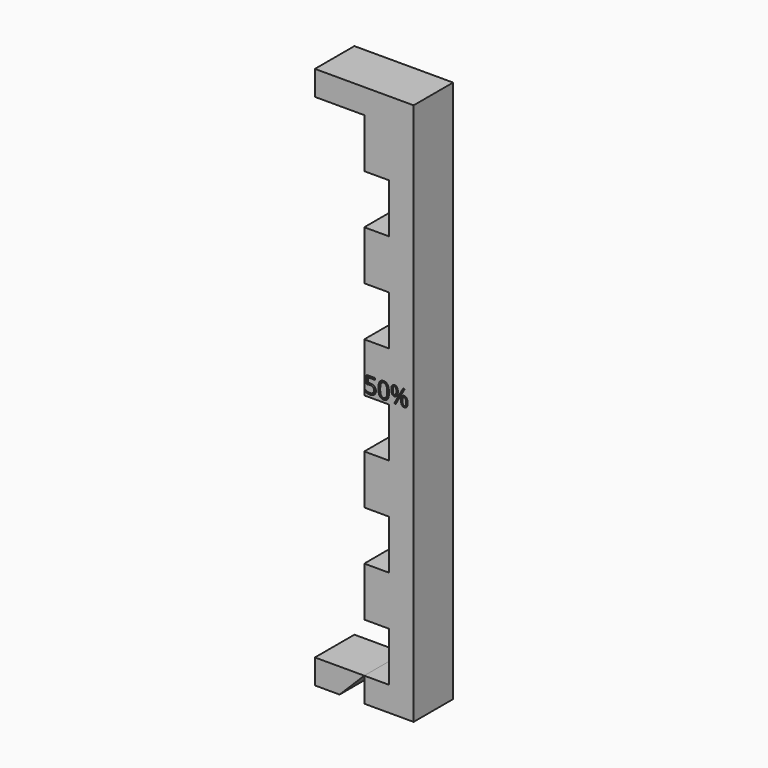
from build123d import *

# Parameters (mm, degrees)
F1_DEPTH     = 110
F2_W         = 10
F2_H         = 10
F3_DEPTH     = 5
F4_SIZE      = 4.99999
F6_DEPTH     = 10
F7_W         = 15
F7_H         = 5
F8_DEPTH     = 10
F9_TEXT_SIZE = 4.5843714191
F10_DEPTH    = 0.5
F11_SCALE    = 0.5
F12_ANGLE    = 90
F13_DEPTH    = 5


# Not quite as in the source:
# - a fillet or chamfer is up to 0.001 mm smaller than in the source, because OpenCascade refuses the exact size
# - Text() gives the source's letters only with a copy of the font that has no kerning and outlines rounded to 1/6400 em; it was checked with that copy


with BuildPart() as f1:
    # F0 (on Front) → F1 (new body)
    with BuildSketch(Plane.XZ):
        Polygon((10, 10), (0, 10), (0, 0), (-10, 0), (-10, -10), (10, -10), align=None)
    extrude(amount=-F1_DEPTH)

    # F5 (on face) → F6 (cut)
    with BuildSketch(Plane.XY.offset(10)):
        Polygon((5, 115), (-10, 115), (-10, 5), (5, 5), (5, 15), (0, 15), (0, 25), (5, 25), (5, 35), (0, 35), (0, 45), (5, 45), (5, 55), (0, 55), (0, 65), (5, 65), (5, 75), (0, 75), (0, 85), (5, 85), (5, 95), (0, 95), (0, 105), (5, 105), align=None)
    extrude(amount=-F6_DEPTH, mode=Mode.SUBTRACT)

    # F7 (on face) → F8 (join)
    with BuildSketch(Plane.XY):
        with Locations((-2.5, 107.5)):
            Rectangle(F7_W, F7_H)
    extrude(amount=F8_DEPTH)

    # F9 (on face) → F10 (cut)
    with BuildSketch(Plane.XY.offset(10)):
        with Locations((0, 55.5388134744)):
            Text('50%', F9_TEXT_SIZE, font='Open Sans', text_align=(TextAlign.LEFT, TextAlign.BOTTOM))
    extrude(amount=-F10_DEPTH, mode=Mode.SUBTRACT)


with BuildPart() as f3:
    # F2 (on face) → F3 (new body)
    with BuildSketch(Plane.XZ):
        with Locations((-5, 5)):
            Rectangle(F2_W, F2_H)
    extrude(amount=-F3_DEPTH)

    # F4 (size 5 in the source; OpenCascade refuses exactly that, so slightly less here)
    f4_edges = [f3.edges().sort_by_distance(p)[0] for p in [
        (0, 0, 5),
    ]]
    chamfer(f4_edges, length=F4_SIZE)


with BuildPart() as f1_1:
    # F11: moved
    add(f1.part.scale(F11_SCALE))


with BuildPart() as f3_1:
    # F11: moved
    add(f3.part.scale(F11_SCALE))


with BuildPart() as f1_2:
    # F12: moved
    add(f1_1.part.rotate(Axis((-2.5, 0, 0), (1, 0, 0)), F12_ANGLE))

    # F13 (cut, through all): a face of the model
    f13_faces = [f1_2.faces().sort_by_distance(p)[0] for p in [
        (0, 5, 27.5),
    ]]
    extrude(f13_faces, amount=-F13_DEPTH, mode=Mode.SUBTRACT)


with BuildPart() as f3_2:
    # F12: moved
    add(f3_1.part.rotate(Axis((-2.5, 0, 0), (1, 0, 0)), F12_ANGLE))


solid = Compound([f1_2.part, f3_2.part])
